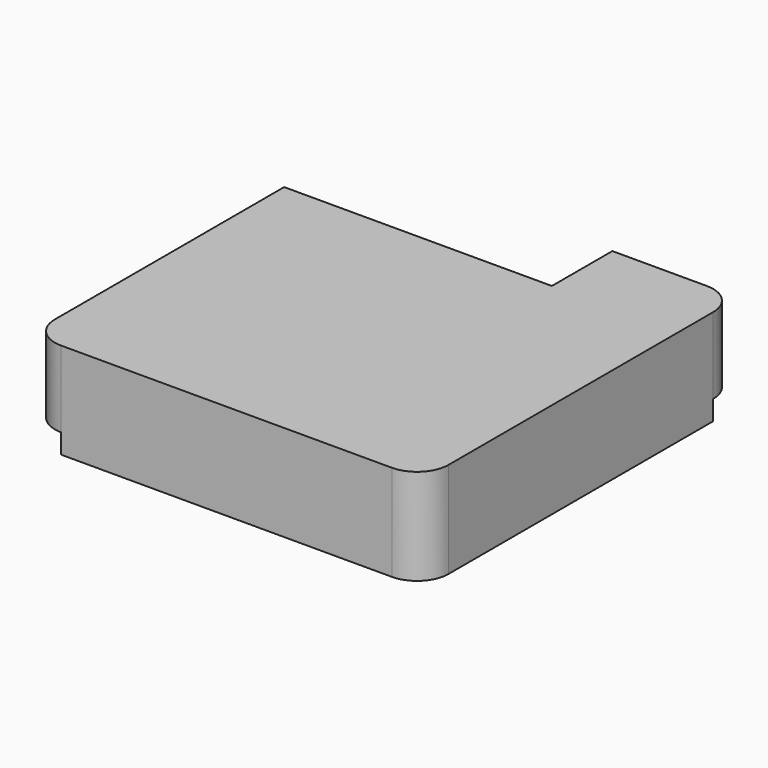
from build123d import *

# Parameters (mm, degrees)
F1_DEPTH = 6.1
F3_DEPTH = 1.25


# Not quite as in the source:
# - a feature names something its author has since deleted; it is built from what else it names


with BuildPart() as f1:
    # F0 (on Top) → F1 (new body)
    with BuildSketch(Plane.XY):
        with BuildLine():
            ThreePointArc((12.5, 10.5), (11.9142135624, 11.9142135624), (10.5, 12.5))
            Line((10.5, 12.5), (4.5, 12.5))
            Line((4.5, 12.5), (4.5, 7.7))
            Line((4.5, 7.7), (-12.5, 7.7))
            Line((-12.5, 7.7), (-12.5, -10.5))
            ThreePointArc((-12.5, -10.5), (-11.9142135624, -11.9142135624), (-10.5, -12.5))
            Line((-10.5, -12.5), (10.5, -12.5))
            ThreePointArc((10.5, -12.5), (11.9142135624, -11.9142135624), (12.5, -10.5))
            Line((12.5, -10.5), (12.5, 10.5))
        make_face()
    extrude(amount=F1_DEPTH)

    # F2 (on face) → F3 (cut)
    with BuildSketch(Plane(origin=(0, 0, 0), x_dir=(1, 0, 0), z_dir=(0, 0, -1))):
        with BuildLine():
            ThreePointArc((10.5, -12.5), (11.9142135624, -11.9142135624), (12.5, -10.5))
            ThreePointArc((12.5, -10.5), (9.0857864376, -9.0857864376), (10.5, -12.5))
        make_face()
        with BuildLine():
            ThreePointArc((-8.5, 10.5), (-9.0857864376, 11.9142135624), (-10.5, 12.5))
            ThreePointArc((-10.5, 12.5), (-11.9142135624, 11.9142135624), (-12.5, 10.5))
            ThreePointArc((-12.5, 10.5), (-10.5, 8.5), (-8.5, 10.5))
        make_face()
    extrude(amount=-F3_DEPTH, mode=Mode.SUBTRACT)


solid = f1.part
